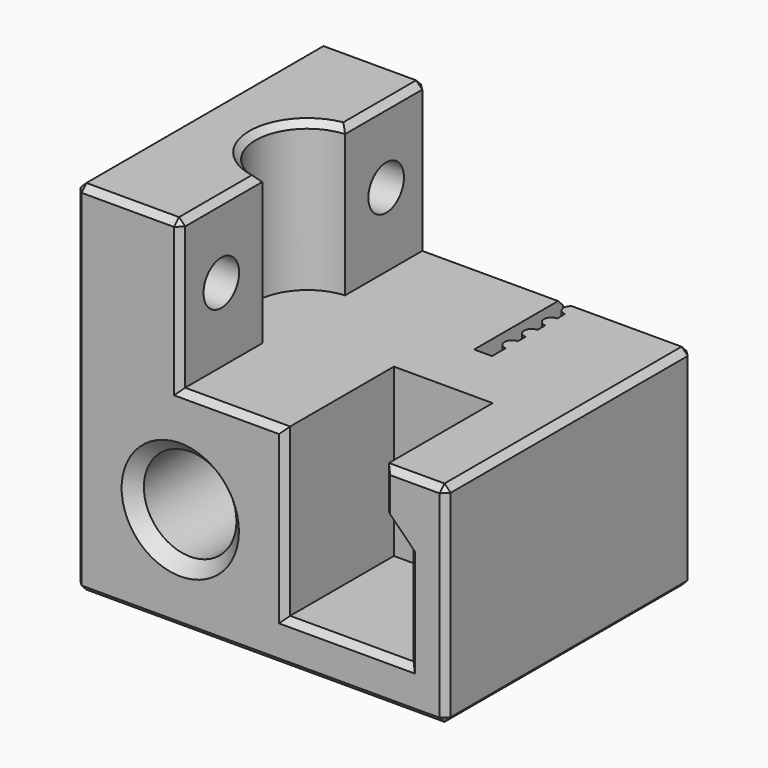
from build123d import *

# Parameters (mm, degrees)
F0_W      = 30
F0_H      = 25
F1_DEPTH  = 17
F3_DEPTH  = 11
F4_R      = 3.75
F5_DEPTH  = 25
F6_W      = 8.5
F6_H      = 25
F7_DEPTH  = 12
F9_DEPTH  = 12
F10_R     = 1.8
F11_DEPTH = 8.5
F12_R     = 1.8
F13_DEPTH = 2.6
F15_DEPTH = 8
F16_R     = 1.8
F17_DEPTH = 14
F18_R     = 1.8
F19_DEPTH = 2.5
F21_SIZE  = 0.5
F22_SIZE2 = 1
F22_SIZE  = 1
F23_R     = 1.35
F24_DEPTH = 5.0024289632


# Not quite as in the source:
# - a feature names something its author has since deleted; it is built from what else it names


with BuildPart() as f1:
    # F0 (on Top) → F1 (new body)
    with BuildSketch(Plane.XY):
        Rectangle(F0_W, F0_H)
    extrude(amount=F1_DEPTH)

    # F2 (on face) → F3 (cut)
    with BuildSketch(Plane.XZ.offset(12.5)):
        Polygon((10, 17), (2, 17), (2, 3.5), (12, 3.5), (12, 11.5), (10, 13.5), align=None)
    extrude(amount=-F3_DEPTH, mode=Mode.SUBTRACT)

    # F4 (on face) → F5 (cut, through all)
    with BuildSketch(Plane.XZ.offset(12.5)):
        with Locations((-6.5, 8.5)):
            Circle(F4_R)
    extrude(amount=-F5_DEPTH, mode=Mode.SUBTRACT)

    # F6 (on face) → F7 (join)
    with BuildSketch(Plane.XY.offset(17)):
        with Locations((-10.75, 0)):
            Rectangle(F6_W, F6_H)
    extrude(amount=F7_DEPTH)

    # F8 (on face) → F9 (cut)
    with BuildSketch(Plane.XY.offset(29)):
        with BuildLine():
            Line((-6.5, -4.1892720131), (-6.5, 4.1892720131))
            ThreePointArc((-6.5, 4.1892720131), (-10.4, 0), (-6.5, -4.1892720131))
        make_face()
    extrude(amount=-F9_DEPTH, mode=Mode.SUBTRACT)

    # F10 (on face) → F11 (cut, through all)
    with BuildSketch(Plane.YZ.offset(-6.5)):
        with Locations((-8.3446360066, 23)):
            Circle(F10_R)
        with Locations((8.3446360066, 23)):
            Circle(F10_R)
    extrude(amount=-F11_DEPTH, mode=Mode.SUBTRACT)

    # F12 (on face) → F13 (cut)
    with BuildSketch(Plane(origin=(-15, 0, 0), x_dir=(0, -1, 0), z_dir=(-1, 0, 0))):
        Polygon((11.3446360067, 21.2679491924), (11.3446360067, 24.7320508076), (8.3446360067, 26.4641016151), (5.3446360067, 24.7320508076), (5.3446360067, 21.2679491924), (8.3446360067, 19.5358983849), align=None)
        with Locations((8.3446360066, 23)):
            Circle(F12_R, mode=Mode.SUBTRACT)
        Polygon((-5.3446360064, 21.2679491924), (-5.3446360064, 24.7320508076), (-8.3446360064, 26.4641016151), (-11.3446360064, 24.7320508076), (-11.3446360064, 21.2679491924), (-8.3446360064, 19.5358983849), align=None)
        with Locations((-8.3446360066, 23)):
            Circle(F12_R, mode=Mode.SUBTRACT)
    extrude(amount=-F13_DEPTH, mode=Mode.SUBTRACT)

    # F14 (on face) → F15 (cut)
    with BuildSketch(Plane.XY.offset(17)):
        with BuildLine():
            Line((5.95, 12.5), (4.5, 12.5))
            Line((4.5, 12.5), (4.5, 3.5))
            Line((4.5, 3.5), (5.95, 3.5))
            Line((5.95, 3.5), (5.95, 4.9))
            ThreePointArc((5.95, 4.9), (5.35, 5.5), (5.95, 6.1))
            Line((5.95, 6.1), (5.95, 6.9))
            ThreePointArc((5.95, 6.9), (5.35, 7.5), (5.95, 8.1))
            Line((5.95, 8.1), (5.95, 8.9))
            ThreePointArc((5.95, 8.9), (5.35, 9.5), (5.95, 10.1))
            Line((5.95, 10.1), (5.95, 10.9))
            ThreePointArc((5.95, 10.9), (5.35, 11.5), (5.95, 12.1))
            Line((5.95, 12.1), (5.95, 12.5))
        make_face()
    extrude(amount=-F15_DEPTH, mode=Mode.SUBTRACT)

    # F16 (on face) → F17 (cut, through all)
    with BuildSketch(Plane(origin=(0, 12.5, 0), x_dir=(-1, 0, 0), z_dir=(0, 1, 0))):
        with Locations((-9.3, 6.5)):
            Circle(F16_R)
    extrude(amount=-F17_DEPTH, mode=Mode.SUBTRACT)

    # F18 (on face) → F19 (cut)
    with BuildSketch(Plane(origin=(0, 12.5, 0), x_dir=(-1, 0, 0), z_dir=(0, 1, 0))):
        Polygon((-7.6256842194, 9.4), (-10.9743157806, 9.4), (-12.6486315613, 6.5), (-10.9743157806, 3.6), (-7.6256842194, 3.6), (-5.9513684387, 6.5), align=None)
        with Locations((-9.3, 6.5)):
            Circle(F18_R, mode=Mode.SUBTRACT)
    extrude(amount=-F19_DEPTH, mode=Mode.SUBTRACT)

    # F21
    f21_edges = [f1.edges().sort_by_distance(p)[0] for p in [
        (0, -12.5, 0),
        (-15, 0, 0),
        (0, 12.5, 0),
        (15, 0, 0),
        (-1, 12.5, 17),
        (10.475, 12.5, 17),
        (-15, 12.5, 14.5),
        (-15, -12.5, 14.5),
        (2, -12.5, 10.25),
        (-6.5, -12.5, 23),
        (7, -12.5, 3.5),
        (12, -12.5, 7.5),
        (11, -12.5, 12.5),
        (10, -12.5, 15.25),
        (15, -12.5, 8.5),
        (12.5, -12.5, 17),
        (15, 0, 17),
        (15, 12.5, 8.5),
        (-6.5, 12.5, 23),
        (-10.75, 12.5, 29),
        (-6.5, 8.344636, 29),
        (-6.5, -8.344636, 29),
        (-10.75, -12.5, 29),
        (-2.25, -12.5, 17),
        (-15, 0, 29),
        (-10.4, 0, 29),
    ]]
    chamfer(f21_edges, length=F21_SIZE)

    # F22
    f22_edges = [f1.edges().sort_by_distance(p)[0] for p in [
        (-2.75, 0, 8.5),
        (-10.25, -12.5, 8.5),
        (-10.25, 12.5, 8.5),
    ]]
    chamfer(f22_edges, length=F22_SIZE, length2=F22_SIZE2)

    # F23 (on face) → F24 (cut, through all)
    with BuildSketch(Plane(origin=(0, 0, 0), x_dir=(1, 0, 0), z_dir=(0, 0, -1))):
        with Locations((-6.5, 0)):
            Circle(F23_R)
    extrude(amount=-F24_DEPTH, mode=Mode.SUBTRACT)


solid = f1.part
